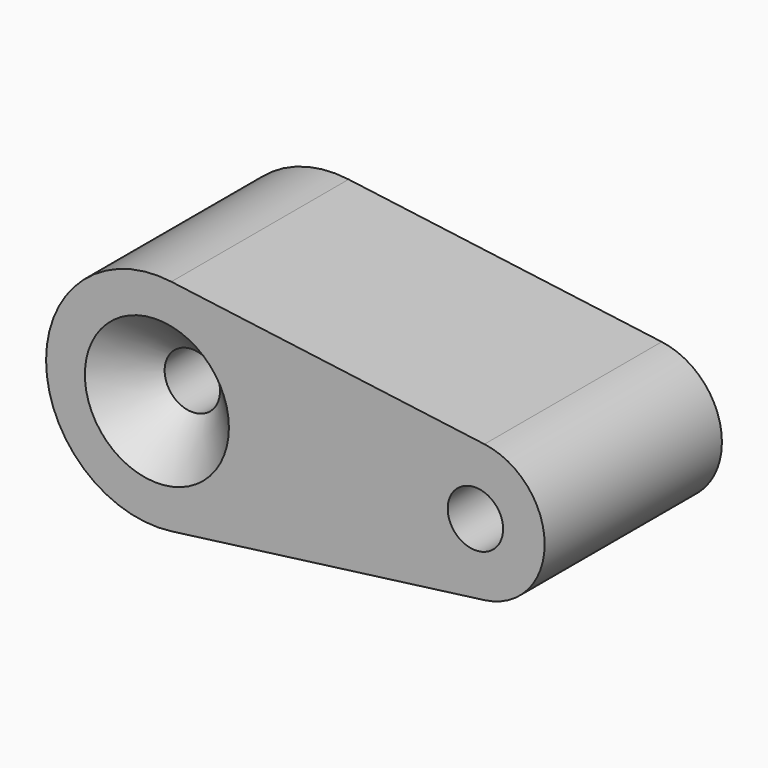
from build123d import *

# Parameters (mm, degrees)
F0_W     = 93.4863612056
F0_H     = 177.5486841798
F0_R     = 7.3874991458
F1_DEPTH = 25.4
F5_R     = 3.175
F6_DEPTH = 25.4
F7_SIZE  = 5.08


# Not quite as in the source:
# - a feature names something its author has since deleted; it is built from what else it names
# - the program builds the solid bodies; features that only make, move or delete a surface that nothing else refers to are left out


with BuildPart() as f1:
    # F0 (on Front) → F1 (new body)
    with BuildSketch(Plane.XZ):
        with Locations((0.2827197313, -1.319359988)):
            Rectangle(F0_W, F0_H)
        Circle(F0_R, mode=Mode.SUBTRACT)
    extrude(amount=F1_DEPTH)


with BuildPart() as f6:
    # F5 (on Front) → F6 (new body)
    with BuildSketch(Plane.XZ):
        with BuildLine():
            ThreePointArc((1.6565217391, -12.5915025207), (9.5479795268, -8.3741320121), (12.7, 0))
            ThreePointArc((12.7, 0), (9.5479795268, 8.3741320121), (1.6565217391, 12.5915025207))
            ThreePointArc((1.6565217391, 12.5915025207), (-12.7, 0), (1.6565217391, -12.5915025207))
        make_face()
        Circle(F5_R, mode=Mode.SUBTRACT)
        with BuildLine():
            ThreePointArc((1.6565217391, 12.5915025207), (9.5479795268, 8.3741320121), (12.7, 0))
            ThreePointArc((12.7, 0), (9.5479795268, -8.3741320121), (1.6565217391, -12.5915025207))
            Line((1.6565217391, -12.5915025207), (37.547826087, -7.8696890754))
            ThreePointArc((37.547826087, -7.8696890754), (28.575, 0), (37.547826087, 7.8696890754))
            Line((37.547826087, 7.8696890754), (1.6565217391, 12.5915025207))
        make_face()
        with BuildLine():
            ThreePointArc((44.45, 0), (42.4799872042, 5.2338325076), (37.547826087, 7.8696890754))
            ThreePointArc((37.547826087, 7.8696890754), (28.575, 0), (37.547826087, -7.8696890754))
            ThreePointArc((37.547826087, -7.8696890754), (42.4799872042, -5.2338325076), (44.45, 0))
        make_face()
        with Locations((36.5125, 0)):
            Circle(F5_R, mode=Mode.SUBTRACT)
    extrude(amount=F6_DEPTH)

    # F7
    f7_edges = [f6.edges().sort_by_distance(p)[0] for p in [
        (-3.175, -25.4, 0),
    ]]
    chamfer(f7_edges, length=F7_SIZE)


solid = f6.part
